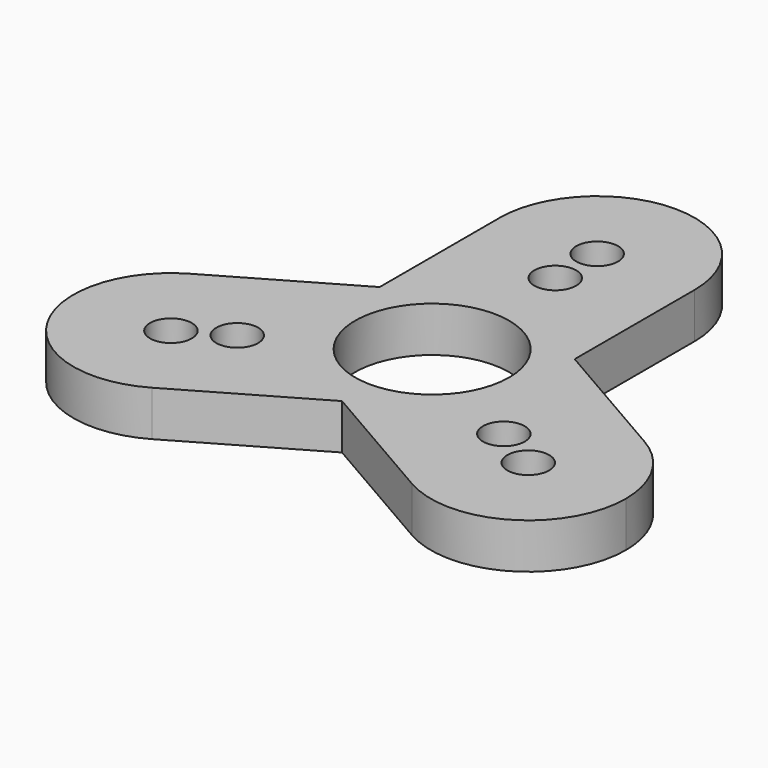
from build123d import *

# Parameters (mm, degrees)
F0_R     = 3
F0_R_2   = 11.05
F1_DEPTH = 6.5


with BuildPart() as f1:
    # F0 (on Top) → F1 (new body)
    with BuildSketch(Plane.XY):
        with BuildLine():
            ThreePointArc((-32.6519768305, -2.6858200754), (-37.7763321694, -21.8101758986), (-18.6519763031, -26.9345310768))
            ThreePointArc((-18.6519763031, -26.9345310768), (-13.5276209102, -21.8101754521), (-11.6519766687, -14.8101756349))
            ThreePointArc((-11.6519766687, -14.8101756349), (-18.6519767496, -2.6858199352), (-32.6519768305, -2.6858200754))
        make_face()
        with Locations((-25.6519766687, -14.8101756349)):
            Circle(F0_R, mode=Mode.SUBTRACT)
        with Locations((-19.1362317873, -11.0483085737)):
            Circle(F0_R, mode=Mode.SUBTRACT)
        with BuildLine():
            Line((0, -16.1658075373), (-7, -12.124355653))
            ThreePointArc((-7, -12.124355653), (-12.124355653, -7), (-14, 0))
            Line((-14, 0), (-14, 8.0829037687))
            Line((-14, 8.0829037687), (-32.6519768305, -2.6858200754))
            ThreePointArc((-32.6519768305, -2.6858200754), (-18.6519767496, -2.6858199352), (-11.6519766687, -14.8101756349))
            ThreePointArc((-11.6519766687, -14.8101756349), (-13.5276209102, -21.8101754521), (-18.6519763031, -26.9345310768))
            Line((-18.6519763031, -26.9345310768), (0, -16.1658075373))
        make_face()
        with BuildLine():
            Line((0, -16.1658075373), (7, -12.124355653))
            ThreePointArc((7, -12.124355653), (0, -14), (-7, -12.124355653))
            Line((-7, -12.124355653), (0, -16.1658075373))
        make_face()
        with BuildLine():
            ThreePointArc((39.6519766687, -14.8101756349), (37.7763323684, -7.8101757158), (32.6519768305, -2.6858200754))
            ThreePointArc((32.6519768305, -2.6858200754), (13.5276209927, -7.8101756747), (18.6519769101, -26.9345314273))
            ThreePointArc((18.6519769101, -26.9345314273), (32.6519767894, -26.9345312182), (39.6519766687, -14.8101756349))
        make_face()
        with Locations((19.1362317873, -11.0483085737)):
            Circle(F0_R, mode=Mode.SUBTRACT)
        with Locations((25.6519766687, -14.8101756349)):
            Circle(F0_R, mode=Mode.SUBTRACT)
        with BuildLine():
            Line((14, 8.0829037687), (14, 0))
            ThreePointArc((14, 0), (12.124355653, -7), (7, -12.124355653))
            Line((7, -12.124355653), (0, -16.1658075373))
            Line((0, -16.1658075373), (18.6519769101, -26.9345314273))
            ThreePointArc((18.6519769101, -26.9345314273), (13.5276209927, -7.8101756747), (32.6519768305, -2.6858200754))
            Line((32.6519768305, -2.6858200754), (14, 8.0829037687))
        make_face()
        with BuildLine():
            ThreePointArc((-14, 29.6203512698), (0, 15.6203512698), (14, 29.6203512698))
            ThreePointArc((14, 29.6203512698), (0, 43.6203512698), (-14, 29.6203512698))
        make_face()
        with Locations((0, 22.0966171473)):
            Circle(F0_R, mode=Mode.SUBTRACT)
        with Locations((0, 29.6203512698)):
            Circle(F0_R, mode=Mode.SUBTRACT)
        with BuildLine():
            ThreePointArc((-7, 12.124355653), (0, 14), (7, 12.124355653))
            Line((7, 12.124355653), (14, 8.0829037687))
            Line((14, 8.0829037687), (14, 29.6203512698))
            ThreePointArc((14, 29.6203512698), (0, 15.6203512698), (-14, 29.6203512698))
            Line((-14, 29.6203512698), (-14, 8.0829037687))
            Line((-14, 8.0829037687), (-7, 12.124355653))
        make_face()
        with BuildLine():
            ThreePointArc((-14, 0), (-12.124355653, 7), (-7, 12.124355653))
            Line((-7, 12.124355653), (-14, 8.0829037687))
            Line((-14, 8.0829037687), (-14, 0))
        make_face()
        with BuildLine():
            ThreePointArc((7, -12.124355653), (12.124355653, -7), (14, 0))
            ThreePointArc((14, 0), (12.124355653, 7), (7, 12.124355653))
            ThreePointArc((7, 12.124355653), (0, 14), (-7, 12.124355653))
            ThreePointArc((-7, 12.124355653), (-12.124355653, 7), (-14, 0))
            ThreePointArc((-14, 0), (-12.124355653, -7), (-7, -12.124355653))
            ThreePointArc((-7, -12.124355653), (0, -14), (7, -12.124355653))
        make_face()
        Circle(F0_R_2, mode=Mode.SUBTRACT)
        with BuildLine():
            ThreePointArc((7, 12.124355653), (12.124355653, 7), (14, 0))
            Line((14, 0), (14, 8.0829037687))
            Line((14, 8.0829037687), (7, 12.124355653))
        make_face()
    extrude(amount=F1_DEPTH)


solid = f1.part
